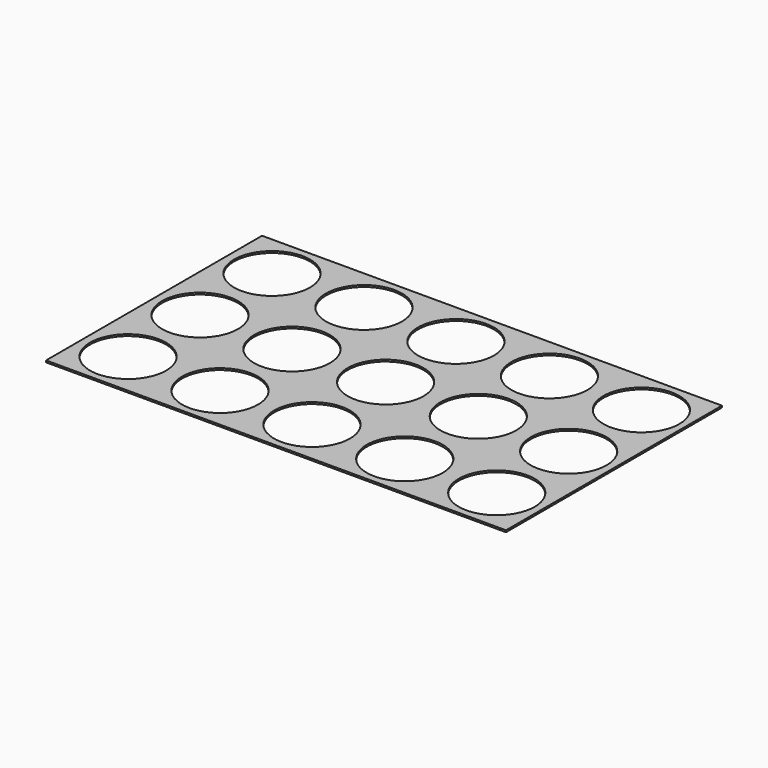
from build123d import *

# Parameters (mm, degrees)
F0_R     = 19
F0_R_2   = 2.5
F1_DEPTH = 0.9
F3_DEPTH = 0.9


# Not quite as in the source:
# - the program builds the solid bodies; features that only make, move or delete a surface that nothing else refers to are left out


with BuildPart() as f1:
    # F0 (on Top) → F1 (new body)
    with BuildSketch(Plane.XY):
        Polygon((127.4130453914, 50.6848765003), (-102.5869546086, 50.6848765003), (-102.5869546086, 5.6848765003), (-102.5869546086, -39.3151234997), (-102.5869546086, -84.3151234997), (-56.5869546086, -84.3151234997), (-10.5869546086, -84.3151234997), (35.4130453914, -84.3151234997), (81.4130453914, -84.3151234997), (127.4130453914, -84.3151234997), align=None)
        with Locations((-79.5869546086, -61.8151234997)):
            Circle(F0_R, mode=Mode.SUBTRACT)
        with Locations((-33.5869546086, -61.8151234997)):
            Circle(F0_R, mode=Mode.SUBTRACT)
        with Locations((12.4130453914, -61.8151234997)):
            Circle(F0_R, mode=Mode.SUBTRACT)
        with Locations((-56.5869546086, -39.3151234997)):
            Circle(F0_R_2, mode=Mode.SUBTRACT)
        with Locations((-10.5869546086, -39.3151234997)):
            Circle(F0_R_2, mode=Mode.SUBTRACT)
        with Locations((58.7792091643, -61.8151234997)):
            Circle(F0_R, mode=Mode.SUBTRACT)
        with Locations((104.7792091643, -61.8151234997)):
            Circle(F0_R, mode=Mode.SUBTRACT)
        with Locations((35.4130453914, -39.3151234997)):
            Circle(F0_R_2, mode=Mode.SUBTRACT)
        with Locations((81.4130453914, -39.3151234997)):
            Circle(F0_R_2, mode=Mode.SUBTRACT)
        with Locations((-79.5869546086, -16.8151234997)):
            Circle(F0_R, mode=Mode.SUBTRACT)
        with Locations((-56.5869546086, 5.6848765003)):
            Circle(F0_R_2, mode=Mode.SUBTRACT)
        with Locations((-33.5869546086, -16.8151234997)):
            Circle(F0_R, mode=Mode.SUBTRACT)
        with Locations((12.4130453914, -15.8099713178)):
            Circle(F0_R, mode=Mode.SUBTRACT)
        with Locations((-10.5869546086, 5.6848765003)):
            Circle(F0_R_2, mode=Mode.SUBTRACT)
        with Locations((-79.5869546086, 28.1848765003)):
            Circle(F0_R, mode=Mode.SUBTRACT)
        with Locations((-33.5869546086, 28.1848765003)):
            Circle(F0_R, mode=Mode.SUBTRACT)
        with Locations((12.4130453914, 28.1848765003)):
            Circle(F0_R, mode=Mode.SUBTRACT)
        with Locations((58.7792091643, -15.8099713178)):
            Circle(F0_R, mode=Mode.SUBTRACT)
        with Locations((35.4130453914, 5.6848765003)):
            Circle(F0_R_2, mode=Mode.SUBTRACT)
        with Locations((104.7792091643, -16.8151234997)):
            Circle(F0_R, mode=Mode.SUBTRACT)
        with Locations((81.4130453914, 5.6848765003)):
            Circle(F0_R_2, mode=Mode.SUBTRACT)
        with Locations((59.1453729371, 28.1848765003)):
            Circle(F0_R, mode=Mode.SUBTRACT)
        with Locations((105.1453729371, 28.1848765003)):
            Circle(F0_R, mode=Mode.SUBTRACT)
    extrude(amount=F1_DEPTH)

    # F0 (on Top) → F3 (join)
    with BuildSketch(Plane.XY):
        with Locations((35.4130453914, -39.3151234997)):
            Circle(F0_R_2)
        with Locations((81.4130453914, -39.3151234997)):
            Circle(F0_R_2)
        with Locations((81.4130453914, 5.6848765003)):
            Circle(F0_R_2)
        with Locations((35.4130453914, 5.6848765003)):
            Circle(F0_R_2)
        with Locations((-10.5869546086, 5.6848765003)):
            Circle(F0_R_2)
        with Locations((-56.5869546086, 5.6848765003)):
            Circle(F0_R_2)
        with Locations((-56.5869546086, -39.3151234997)):
            Circle(F0_R_2)
        with Locations((-10.5869546086, -39.3151234997)):
            Circle(F0_R_2)
    extrude(amount=F3_DEPTH)


solid = f1.part
